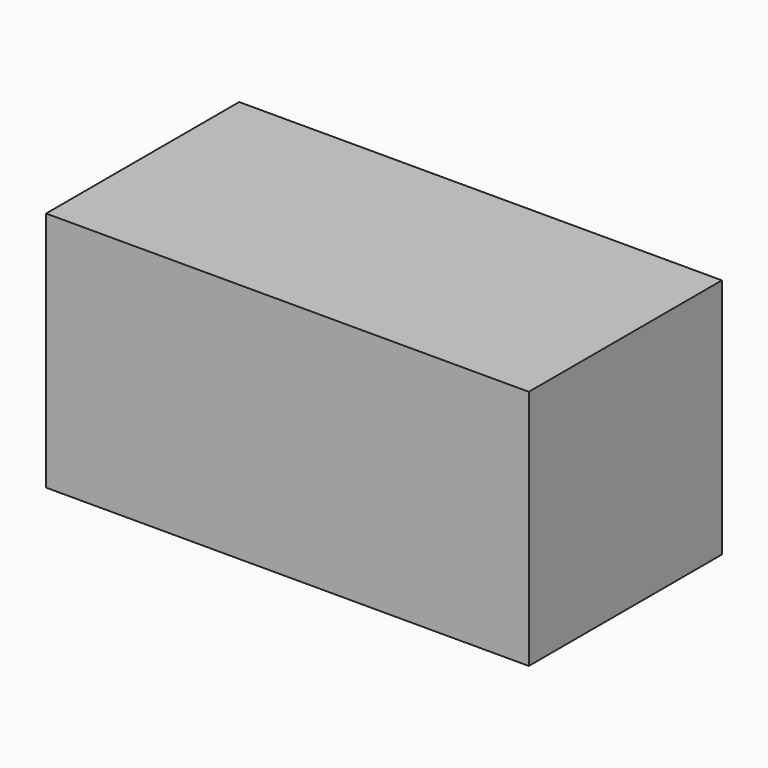
from build123d import *

# Parameters (mm, degrees)
F0_W     = 101.6
F0_H     = 50.8
F1_DEPTH = 25.4


# Not quite as in the source:
# - a feature names something its author has since deleted; it is built from what else it names


with BuildPart() as f1:
    # F0 (on Front) → F1 (new body, symmetric)
    with BuildSketch(Plane.XZ):
        with Locations((25.4, 0)):
            Rectangle(F0_W, F0_H)
    extrude(amount=F1_DEPTH, both=True)


solid = f1.part
